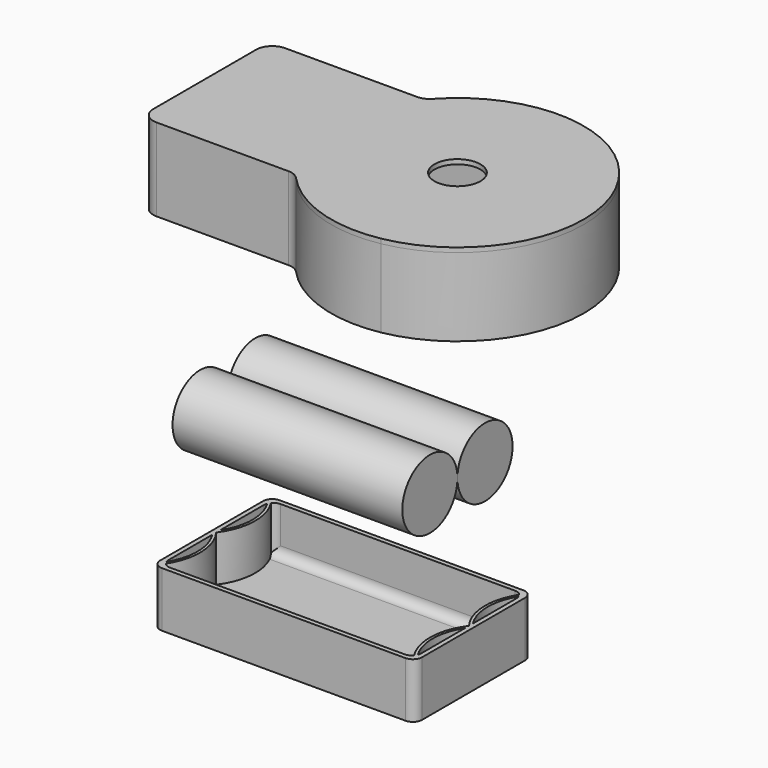
from build123d import *

# Parameters (mm, degrees)
F0_W      = 57
F0_H      = 32
F0_W_2    = 55
F0_H_2    = 30
F1_DEPTH  = 2
F2_DEPTH  = 10
F3_R      = 2
F4_R      = 7.5
F5_DEPTH  = 25
F7_DEPTH  = 10
F10_DEPTH = 1
F11_DEPTH = 17


# Not quite as in the source:
# - a feature names something its author has since deleted; it is built from what else it names


with BuildPart() as f1:
    # F0 (on Top) → F1 (new body)
    with BuildSketch(Plane.XY):
        Rectangle(F0_W, F0_H)
        Rectangle(F0_W_2, F0_H_2, mode=Mode.SUBTRACT)
        Rectangle(F0_W_2, F0_H_2)
    extrude(amount=-F1_DEPTH)

    # F0 (on Top) → F2 (join)
    with BuildSketch(Plane.XY):
        Rectangle(F0_W, F0_H)
        Rectangle(F0_W_2, F0_H_2, mode=Mode.SUBTRACT)
    extrude(amount=F2_DEPTH)

    # F3
    f3_edges = [f1.edges().sort_by_distance(p)[0] for p in [
        (-27.5, 15, 5),
        (-28.5, 16, 4),
        (-27.5, -15, 5),
        (28.5, 16, 4),
        (-28.5, -16, 4),
        (27.5, 15, 5),
        (27.5, -15, 5),
        (28.5, -16, 4),
        (0, 15, 0),
        (0, -15, 0),
    ]]
    fillet(f3_edges, radius=F3_R)

    # F6 (on Top) → F7 (join)
    with BuildSketch(Plane.XY):
        with BuildLine():
            Line((-27.5, 1.0494186309), (-27.5, 0))
            ThreePointArc((-27.5, 0), (-25, 7.5), (-27.5, 15))
            Line((-27.5, 15), (-27.5, 13.9505813691))
            ThreePointArc((-27.5, 13.9505813691), (-25.6, 7.5), (-27.5, 1.0494186309))
        make_face()
        with BuildLine():
            ThreePointArc((-27.5, -15), (-25, -7.5), (-27.5, 0))
            Line((-27.5, 0), (-27.5, -1.0494186309))
            ThreePointArc((-27.5, -1.0494186309), (-25.6, -7.5), (-27.5, -13.9505813691))
            Line((-27.5, -13.9505813691), (-27.5, -15))
        make_face()
        with BuildLine():
            ThreePointArc((27.5, 15), (25, 7.5), (27.5, 0))
            Line((27.5, 0), (27.5, 1.0494186309))
            ThreePointArc((27.5, 1.0494186309), (25.6, 7.5), (27.5, 13.9505813691))
            Line((27.5, 13.9505813691), (27.5, 15))
        make_face()
        with BuildLine():
            ThreePointArc((27.5, -13.9505813691), (25.6, -7.5), (27.5, -1.0494186309))
            Line((27.5, -1.0494186309), (27.5, 0))
            ThreePointArc((27.5, 0), (25, -7.5), (27.5, -15))
            Line((27.5, -15), (27.5, -13.9505813691))
        make_face()
    extrude(amount=F7_DEPTH)


with BuildPart() as f5:
    # F4 (on Right) → F5 (new body, symmetric)
    with BuildSketch(Plane.YZ):
        with Locations((-7.5, 7.5)):
            Circle(F4_R)
    extrude(amount=F5_DEPTH, both=True)


with BuildPart() as f5b:
    # F4 (on Right) → F5, piece 2 (new body, symmetric)
    with BuildSketch(Plane.YZ):
        with BuildLine():
            ThreePointArc((15, 7.5), (7.5, 15), (0, 7.5))
            ThreePointArc((0, 7.5), (7.5, 0), (15, 7.5))
        make_face()
    extrude(amount=F5_DEPTH, both=True)


with BuildPart() as f10:
    # F9 (on offset) → F10 (new body)
    with BuildSketch(Plane.XY.offset(15)):
        with BuildLine():
            Line((30, -27.0416345442), (30, 0))
            Line((30, 0), (30, 27.0416345442))
            ThreePointArc((30, 27.0416345442), (16.3009792126, 26.0878714998), (4.7710810497, 18.6290322581))
            ThreePointArc((4.7710810497, 18.6290322581), (3.6021252057, 17.7946617108), (2.1964913802, 17.5))
            Line((2.1964913802, 17.5), (-26.5, 17.5))
            ThreePointArc((-26.5, 17.5), (-28.9748737342, 16.4748737342), (-30, 14))
            Line((-30, 14), (-30, -14))
            ThreePointArc((-30, -14), (-28.9748737342, -16.4748737342), (-26.5, -17.5))
            Line((-26.5, -17.5), (2.1964913802, -17.5))
            ThreePointArc((2.1964913802, -17.5), (3.6021252057, -17.7946617108), (4.7710810497, -18.6290322581))
            ThreePointArc((4.7710810497, -18.6290322581), (16.3009792126, -26.0878714998), (30, -27.0416345442))
        make_face()
        with BuildLine():
            ThreePointArc((29, -14), (28.267766953, -15.767766953), (26.5, -16.5))
            Line((26.5, -16.5), (-26.5, -16.5))
            ThreePointArc((-26.5, -16.5), (-28.267766953, -15.767766953), (-29, -14))
            Line((-29, -14), (-29, 14))
            ThreePointArc((-29, 14), (-28.267766953, 15.767766953), (-26.5, 16.5))
            Line((-26.5, 16.5), (26.5, 16.5))
            ThreePointArc((26.5, 16.5), (28.267766953, 15.767766953), (29, 14))
            Line((29, 14), (29, 2.9999998428))
            ThreePointArc((29, 2.9999998428), (29.7434164034, 1.5811387369), (29.9999998821, 0))
            ThreePointArc((29.9999998821, 0), (29.7434164034, -1.5811387369), (29, -2.9999998428))
            Line((29, -2.9999998428), (29, -14))
        make_face(mode=Mode.SUBTRACT)
        with BuildLine():
            Line((-26.5, -16.5), (26.5, -16.5))
            ThreePointArc((26.5, -16.5), (28.267766953, -15.767766953), (29, -14))
            Line((29, -14), (29, -2.9999998428))
            ThreePointArc((29, -2.9999998428), (19.9999998821, 0), (29, 2.9999998428))
            Line((29, 2.9999998428), (29, 14))
            ThreePointArc((29, 14), (28.267766953, 15.767766953), (26.5, 16.5))
            Line((26.5, 16.5), (-26.5, 16.5))
            ThreePointArc((-26.5, 16.5), (-28.267766953, 15.767766953), (-29, 14))
            Line((-29, 14), (-29, -14))
            ThreePointArc((-29, -14), (-28.267766953, -15.767766953), (-26.5, -16.5))
        make_face()
        with BuildLine():
            Line((30, 27.0416345442), (30, 0))
            Line((30, 0), (30, -27.0416345442))
            ThreePointArc((30, -27.0416345442), (52.4999998821, 0), (30, 27.0416345442))
        make_face()
    extrude(amount=F10_DEPTH)

    # F9 (on offset) → F11 (join)
    with BuildSketch(Plane.XY.offset(15)):
        with BuildLine():
            Line((30, -27.0416345442), (30, 0))
            Line((30, 0), (30, 27.0416345442))
            ThreePointArc((30, 27.0416345442), (16.3009792126, 26.0878714998), (4.7710810497, 18.6290322581))
            ThreePointArc((4.7710810497, 18.6290322581), (3.6021252057, 17.7946617108), (2.1964913802, 17.5))
            Line((2.1964913802, 17.5), (-26.5, 17.5))
            ThreePointArc((-26.5, 17.5), (-28.9748737342, 16.4748737342), (-30, 14))
            Line((-30, 14), (-30, -14))
            ThreePointArc((-30, -14), (-28.9748737342, -16.4748737342), (-26.5, -17.5))
            Line((-26.5, -17.5), (2.1964913802, -17.5))
            ThreePointArc((2.1964913802, -17.5), (3.6021252057, -17.7946617108), (4.7710810497, -18.6290322581))
            ThreePointArc((4.7710810497, -18.6290322581), (16.3009792126, -26.0878714998), (30, -27.0416345442))
        make_face()
        with BuildLine():
            ThreePointArc((29, -14), (28.267766953, -15.767766953), (26.5, -16.5))
            Line((26.5, -16.5), (-26.5, -16.5))
            ThreePointArc((-26.5, -16.5), (-28.267766953, -15.767766953), (-29, -14))
            Line((-29, -14), (-29, 14))
            ThreePointArc((-29, 14), (-28.267766953, 15.767766953), (-26.5, 16.5))
            Line((-26.5, 16.5), (26.5, 16.5))
            ThreePointArc((26.5, 16.5), (28.267766953, 15.767766953), (29, 14))
            Line((29, 14), (29, 2.9999998428))
            ThreePointArc((29, 2.9999998428), (29.7434164034, 1.5811387369), (29.9999998821, 0))
            ThreePointArc((29.9999998821, 0), (29.7434164034, -1.5811387369), (29, -2.9999998428))
            Line((29, -2.9999998428), (29, -14))
        make_face(mode=Mode.SUBTRACT)
        with BuildLine():
            Line((30, 27.0416345442), (30, 0))
            Line((30, 0), (30, -27.0416345442))
            ThreePointArc((30, -27.0416345442), (52.4999998821, 0), (30, 27.0416345442))
        make_face()
        with BuildLine():
            Line((29, 2.9999998428), (29, -2.9999998428))
            ThreePointArc((29, -2.9999998428), (29.7434164034, -1.5811387369), (29.9999998821, 0))
            ThreePointArc((29.9999998821, 0), (29.7434164034, 1.5811387369), (29, 2.9999998428))
        make_face()
    extrude(amount=-F11_DEPTH)


with BuildPart() as f10_1:
    # F12: moved
    add(f10.part.moved(Location((0, 0, 50))))


with BuildPart() as f1_1:
    # F13: moved
    add(f1.part.moved(Location((0, 0, -30))))


solid = Compound([f5.part, f5b.part, f10_1.part, f1_1.part])
